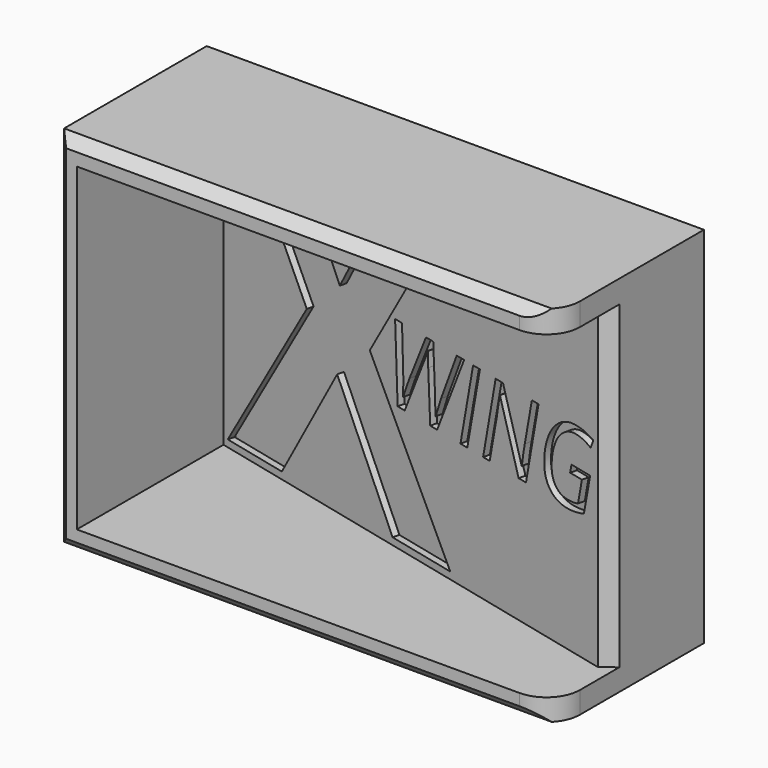
from build123d import *

# Parameters (mm, degrees)
F1_DEPTH     = 28
F3_DEPTH     = 54
F4_SIZE      = 1.5
F5_R         = 5
F6_SIZE      = 2
F8_TEXT_SIZE = 15.742248959
F9_DEPTH     = 1
F7_TEXT_SIZE = 63.0851899688
F10_DEPTH    = 1


# Not quite as in the source:
# - Text() gives the source's letters only with a copy of the font that has no kerning and outlines rounded to 1/6400 em; it was checked with that copy


with BuildPart() as f1:
    # F0 (on Front) → F1 (new body)
    with BuildSketch(Plane.XZ):
        Polygon((-42.8640022874, 0), (31.0588441789, 0), (31.0588441789, 3.2323680352), (-39.7721715271, 3.2323680352), (-39.7721715271, 50.7341250777), (31.0588441789, 50.7341250777), (31.0588441789, 54.107028991), (-42.8640022874, 54.107028991), align=None)
    extrude(amount=-F1_DEPTH)

    # F2 (on face) → F3 (join)
    with BuildSketch(Plane(origin=(0, 0, 0), x_dir=(1, 0, 0), z_dir=(0, 0, -1))):
        Polygon((31.0588441789, -10.2894175798), (-42.8640022874, -28), (31.0588441789, -28), align=None)
    extrude(amount=-F3_DEPTH)

    # F4
    f4_edges = [f1.edges().sort_by_distance(p)[0] for p in [
        (-5.902579, 0, 0),
        (-42.864002, 0, 27.053514),
        (-5.902579, 0, 54.107029),
    ]]
    chamfer(f4_edges, length=F4_SIZE)

    # F5
    f5_edges = [f1.edges().sort_by_distance(p)[0] for p in [
        (31.058844, 0, 51.670577),
        (31.058844, 0, 2.366184),
    ]]
    fillet(f5_edges, radius=F5_R)

    # F6
    f6_edges = [f1.edges().sort_by_distance(p)[0] for p in [
        (31.058844, 10.289418, 26.983247),
    ]]
    chamfer(f6_edges, length=F6_SIZE)

    # F8 (on face) → F9 (cut)
    with BuildSketch(Plane(origin=(4.0173293058, 16.7680774369, 0), x_dir=(0.9724794747, -0.2329885646, 0), z_dir=(-0.2329885646, -0.9724794747, 0))):
        with Locations((-14.2865683883, 21.7988733202)):
            Text('WING', F8_TEXT_SIZE, font='Open Sans', font_style=FontStyle.ITALIC, text_align=(TextAlign.LEFT, TextAlign.BOTTOM))
    extrude(amount=-F9_DEPTH, mode=Mode.SUBTRACT)

    # F7 (on face) → F10 (cut)
    with BuildSketch(Plane(origin=(4.0173293058, 16.7680774369, 0), x_dir=(0.9724794747, -0.2329885646, 0), z_dir=(-0.2329885646, -0.9724794747, 0))):
        with Locations((-44.2221397534, 4.2632771656)):
            Text('X', F7_TEXT_SIZE, font='Open Sans', font_style=FontStyle.BOLD, text_align=(TextAlign.LEFT, TextAlign.BOTTOM))
    extrude(amount=-F10_DEPTH, mode=Mode.SUBTRACT)


solid = f1.part
